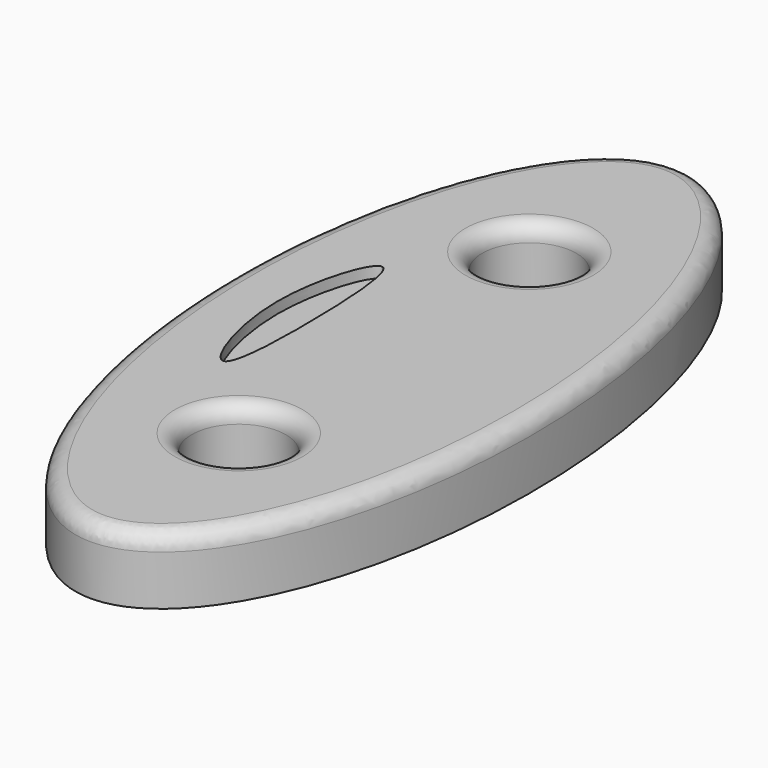
from build123d import *

# Parameters (mm, degrees)
F1_DEPTH = 3.048
F2_R     = 2.159
F3_DEPTH = 25.4
F5_DEPTH = 25.4
F6_R     = 0.762
F8_DEPTH = 0.508


with BuildPart() as f1:
    # F0 (on Top) → F1 (new body)
    with BuildSketch(Plane.XY):
        with BuildLine():
            add(Edge.make_bspline(
                [(0.6613530173, -17.4499718749), (13.9436895104, -16.9465720196), (6.3104917379, 8.9766858651), (-1.3227060347, 34.8999437499), (-6.9718447552, 8.4732860098), (-12.6209834757, -17.9533717302), (0.6613530173, -17.4499718749)],
                knots=[0, 0, 0, 2.0943951024, 2.0943951024, 4.1887902048, 4.1887902048, 6.2831853072, 6.2831853072, 6.2831853072], degree=2, weights=[1, 0.5, 1, 0.5, 1, 0.5, 1]))
        make_face()
    extrude(amount=F1_DEPTH)

    # F2 (on face) → F3 (cut)
    with BuildSketch(Plane.XY.offset(3.048)):
        with Locations((0.3306765087, -8.7249859375)):
            Circle(F2_R)
    extrude(amount=-F3_DEPTH, mode=Mode.SUBTRACT)

    # F4 (on face) → F5 (cut)
    with BuildSketch(Plane.XY.offset(3.048)):
        with BuildLine():
            ThreePointArc((1.8283234913, 8.7249859375), (1.166778906, 10.2802699247), (-0.4124437908, 10.8824370056))
            Line((-0.4124437908, 10.8824370056), (-0.3306765087, 8.7249859375))
            Line((-0.3306765087, 8.7249859375), (-0.2489092265, 6.5675348693))
            ThreePointArc((-0.2489092265, 6.5675348693), (1.2246074786, 7.2275305228), (1.8283234913, 8.7249859375))
        make_face()
        with BuildLine():
            Line((-0.3306765087, 8.7249859375), (-0.4124437908, 10.8824370056))
            ThreePointArc((-0.4124437908, 10.8824370056), (-2.4881275768, 8.6432186553), (-0.2489092265, 6.5675348693))
            Line((-0.2489092265, 6.5675348693), (-0.3306765087, 8.7249859375))
        make_face()
    extrude(amount=-F5_DEPTH, mode=Mode.SUBTRACT)

    # F6
    f6_edges = [f1.edges().sort_by_distance(p)[0] for p in [
        (-1.828323, -8.724986, 3.048),
        (-0.661344, 17.449972, 3.048),
        (-2.489677, 8.724986, 3.048),
    ]]
    fillet(f6_edges, radius=F6_R)

    # F7 (on face) → F8 (cut)
    with BuildSketch(Plane.XY.offset(3.048)):
        with BuildLine():
            add(Edge.make_bspline(
                [(-3.7330428604, 4.5394091867), (-4.2051300167, 4.5578602615), (-5.7928040731, -0.0081425775), (-3.2125997952, -7.0762809617), (-2.9436366007, 0.0059427831), (-3.2668165411, 4.5211871771), (-3.7330428604, 4.5394091867)],
                knots=[0, 0, 0, 0, 0.2492966101, 0.5037465374, 0.7537983413, 1, 1, 1, 1], degree=3))
        make_face()
    extrude(amount=-F8_DEPTH, mode=Mode.SUBTRACT)


solid = f1.part
